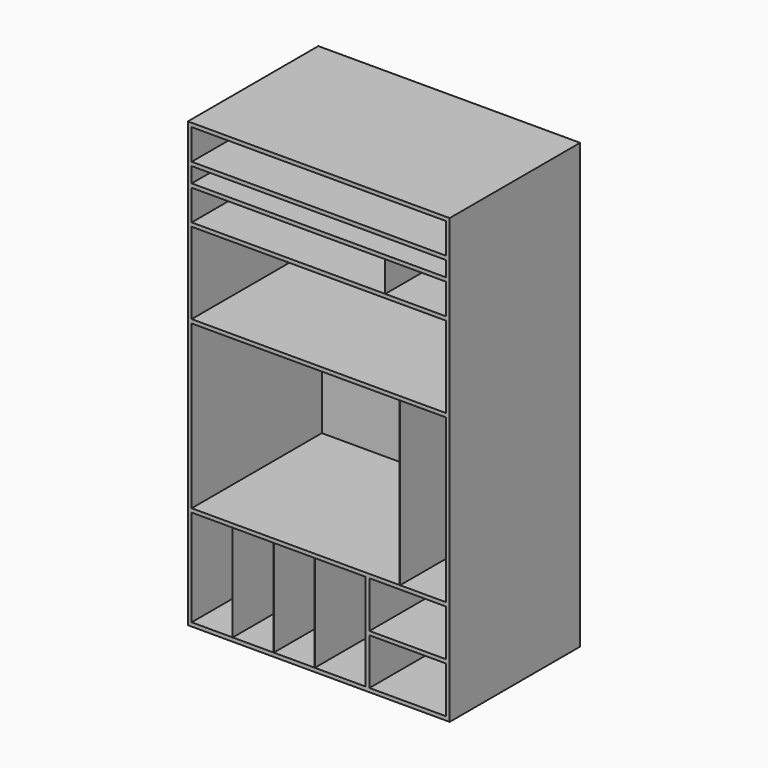
from build123d import *

# Parameters (mm, degrees)
F0_W     = 1270
F0_H     = 19.05
F0_W_2   = 1.905
F0_H_2   = 482.6
F0_H_3   = 152.4
F0_H_4   = 812.8
F0_W_3   = 381.635
F1_DEPTH = 812.8
F3_START = -812.8
F2_W     = 1308.1
F2_H     = 2216.15
F3_DEPTH = 1.905


# Not quite as in the source:
# - a feature names something its author has since deleted; it is built from what else it names


with BuildPart() as f1:
    # F0 (on Front) → F1 (new body)
    with BuildSketch(Plane.XZ):
        Polygon((-635, -396.875), (-635, 415.925), (-635, 434.975), (-635, 841.375), (-635, 860.425), (-635, 1012.825), (-635, 1031.875), (-635, 1108.075), (-635, 1127.125), (-635, 1279.525), (-635, 1298.575), (-654.05, 1298.575), (-654.05, -917.575), (-635, -917.575), (-635, -898.525), (-635, -415.925), align=None)
        Polygon((-635, 434.975), (-635, 415.925), (404.495, 415.925), (406.4, 415.925), (635, 415.925), (635, 434.975), align=None)
        Polygon((-635, 860.425), (-635, 841.375), (635, 841.375), (635, 860.425), (332.105, 860.425), (330.2, 860.425), (0, 860.425), align=None)
        Polygon((-635, 1031.875), (-635, 1012.825), (0, 1012.825), (330.2, 1012.825), (332.105, 1012.825), (635, 1012.825), (635, 1031.875), align=None)
        with Locations((0, 1289.05)):
            Rectangle(F0_W, F0_H)
        Polygon((635, 841.375), (635, 434.975), (635, 415.925), (635, -396.875), (635, -415.925), (635, -647.7), (635, -666.75), (635, -898.525), (635, -917.575), (654.05, -917.575), (654.05, 1298.575), (635, 1298.575), (635, 1279.525), (635, 1127.125), (635, 1108.075), (635, 1031.875), (635, 1012.825), (635, 860.425), align=None)
        Polygon((404.495, -396.875), (-635, -396.875), (-635, -415.925), (-431.8, -415.925), (-429.895, -415.925), (-226.695, -415.925), (-224.79, -415.925), (-21.59, -415.925), (-19.685, -415.925), (234.315, -415.925), (253.365, -415.925), (635, -415.925), (635, -396.875), (406.4, -396.875), align=None)
        Polygon((-431.8, -898.525), (-635, -898.525), (-635, -917.575), (635, -917.575), (635, -898.525), (253.365, -898.525), (234.315, -898.525), (-19.685, -898.525), (-21.59, -898.525), (-224.79, -898.525), (-226.695, -898.525), (-429.895, -898.525), align=None)
        with Locations((-430.8475, -657.225)):
            Rectangle(F0_W_2, F0_H_2)
        with Locations((-225.7425, -657.225)):
            Rectangle(F0_W_2, F0_H_2)
        with Locations((-20.6375, -657.225)):
            Rectangle(F0_W_2, F0_H_2)
        with Locations((0, 1117.6)):
            Rectangle(F0_W, F0_H)
        with Locations((331.1525, 936.625)):
            Rectangle(F0_W_2, F0_H_3)
        with Locations((405.4475, 9.525)):
            Rectangle(F0_W_2, F0_H_4)
        Polygon((253.365, -647.7), (253.365, -415.925), (234.315, -415.925), (234.315, -898.525), (253.365, -898.525), (253.365, -666.75), align=None)
        with Locations((444.1825, -657.225)):
            Rectangle(F0_W_3, F0_H)
    extrude(amount=F1_DEPTH)

    # F2 (on face) → F3 (join)
    with BuildSketch(Plane.XZ.offset(812.8).offset(F3_START)):
        with Locations((0, 190.5)):
            Rectangle(F2_W, F2_H)
    extrude(amount=-F3_DEPTH)


solid = f1.part
